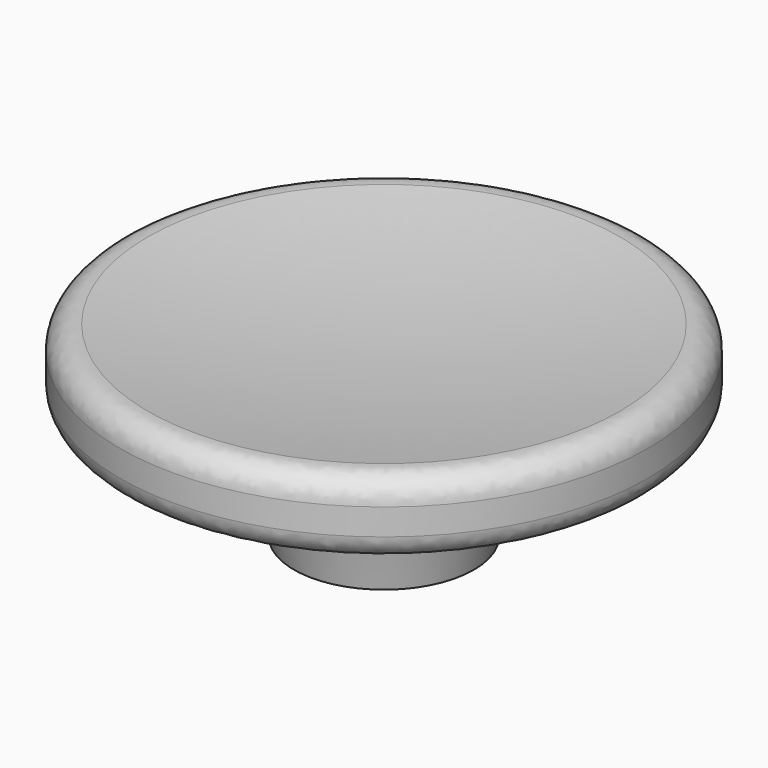
from build123d import *

# Parameters (mm, degrees)
F2_R = 1


# Not quite as in the source:
# - a fillet or chamfer that OpenCascade refuses, or shapes differently, is made with other operations: its cross-section is extruded or revolved along the edge and cut away or added


with BuildPart() as f1:
    # F0 (on Front) → F1 (revolve)
    with BuildSketch(Plane.XZ):
        with BuildLine():
            Line((0, 6.9830484122), (0, 0))
            Line((0, 0), (4.05, 0))
            Line((4.05, 0), (4.05, 3))
            Line((4.05, 3), (5.25, 3))
            Line((5.25, 3), (11, 5))
            Line((11, 5), (11, 8))
            ThreePointArc((11, 8), (5.5234543207, 7.2378272446), (0, 6.9830484122))
        make_face()
    revolve(axis=Axis((0, 0, 1.772551451), (0, 0, 1)))

    # F2
    f2_edges = [f1.edges().sort_by_distance(p)[0] for p in [
        (-11, 0, 5),
        (-11, 0, 8),
    ]]
    fillet(f2_edges, radius=F2_R)

    # F3: chamfer of 0.3 x 1.5 on 1 edges, made by hand

    # F3_s1 → F3_t2 (revolve, cut)
    with BuildSketch(Plane.XZ):
        Polygon((4.05, 1.5), (3.75, 0), (4.05, 0), align=None)
    revolve(axis=Axis((0, 0, 0), (0, 0, 1)), mode=Mode.SUBTRACT)


solid = f1.part
